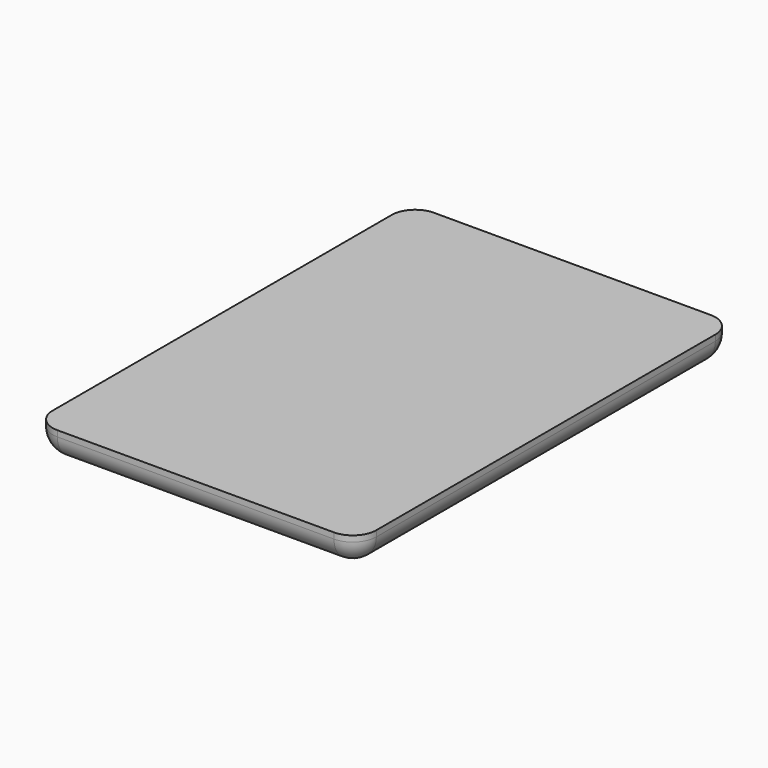
from build123d import *

# Parameters (mm, degrees)
F0_W         = 69.85
F0_H         = 101.6
F1_DEPTH     = 6.35
F2_R         = 5.08
F3_T1_DEPTH  = 13.97
F3_S5_W      = 5.08
F3_S5_H      = 5.08
F3_T6_DEPTH  = 5.08
F3_S11_W     = 5.08
F3_S11_H     = 5.08
F3_T12_DEPTH = 5.08
F3_S17_W     = 5.08
F3_S17_H     = 5.08
F3_T18_DEPTH = 5.08
F3_S23_W     = 5.08
F3_S23_H     = 5.08
F3_T24_DEPTH = 5.08


# Not quite as in the source:
# - a fillet or chamfer that OpenCascade refuses, or shapes differently, is made with other operations: its cross-section is extruded or revolved along the edge and cut away or added


with BuildPart() as f1:
    # F0 (on Top) → F1 (new body)
    with BuildSketch(Plane.XY):
        with Locations((34.925, -50.8)):
            Rectangle(F0_W, F0_H)
    extrude(amount=F1_DEPTH)

    # F2
    f2_edges = [f1.edges().sort_by_distance(p)[0] for p in [
        (69.85, -50.8, 0),
        (34.925, -101.6, 0),
        (0, -50.8, 0),
        (34.925, 0, 0),
    ]]
    fillet(f2_edges, radius=F2_R)

    # F3: fillet of radius 5.08 on 4 edges, made by hand

    # F3_s2 → F3_t1 (cut)
    with BuildSketch(Plane.XY.offset(5.08)):
        with BuildLine():
            ThreePointArc((0, -96.52), (1.4878975516, -100.1121024484), (5.08, -101.6))
            Line((5.08, -101.6), (0, -101.6))
            Line((0, -101.6), (0, -96.52))
        make_face()
        with BuildLine():
            ThreePointArc((64.77, 0), (68.3621024484, -1.4878975516), (69.85, -5.08))
            Line((69.85, -5.08), (69.85, 0))
            Line((69.85, 0), (64.77, 0))
        make_face()
        with BuildLine():
            ThreePointArc((5.08, 0), (1.4878975516, -1.4878975516), (0, -5.08))
            Line((0, -5.08), (0, 0))
            Line((0, 0), (5.08, 0))
        make_face()
        with BuildLine():
            ThreePointArc((69.85, -96.52), (68.3621024484, -100.1121024484), (64.77, -101.6))
            Line((64.77, -101.6), (69.85, -101.6))
            Line((69.85, -101.6), (69.85, -96.52))
        make_face()
    extrude(amount=F3_T1_DEPTH, mode=Mode.SUBTRACT)


with BuildPart() as f3_tool4:
    # F3_s5 → F3_t6 (new body)
    with BuildSketch(Plane.YZ.offset(64.77)):
        with Locations((-99.06, 2.54)):
            Rectangle(F3_S5_W, F3_S5_H)
    extrude(amount=F3_T6_DEPTH)

    # F3_s7 → F3_t8 (revolve, cut)
    with BuildSketch(Plane(origin=(64.77, -96.52, 5.08), x_dir=(0, 0.7071067812, 0.7071067812), z_dir=(0, 0.7071067812, -0.7071067812))):
        with BuildLine():
            ThreePointArc((0, -5.08), (5.08, 0), (0, 5.08))
            Line((0, 5.08), (0, -5.08))
        make_face()
    revolve(axis=Axis((64.77, -96.52, 5.08), (1, 0, 0)), mode=Mode.SUBTRACT)


with BuildPart() as f1_1:
    add(f1.part)

    # F3_t3: cut F3_tool4
    add(f3_tool4.part, mode=Mode.SUBTRACT)


with BuildPart() as f3_tool10:
    # F3_s11 → F3_t12 (new body)
    with BuildSketch(Plane.XZ.offset(5.08)):
        with Locations((2.54, 2.54)):
            Rectangle(F3_S11_W, F3_S11_H)
    extrude(amount=-F3_T12_DEPTH)

    # F3_s13 → F3_t14 (revolve, cut)
    with BuildSketch(Plane(origin=(5.08, -5.08, 5.08), x_dir=(0.7071067812, 0, 0.7071067812), z_dir=(-0.7071067812, 0, 0.7071067812))):
        with BuildLine():
            ThreePointArc((0, -5.08), (5.08, 0), (0, 5.08))
            Line((0, 5.08), (0, -5.08))
        make_face()
    revolve(axis=Axis((5.08, -5.08, 5.08), (0, 1, 0)), mode=Mode.SUBTRACT)


with BuildPart() as f1_2:
    add(f1_1.part)

    # F3_t9: cut F3_tool10
    add(f3_tool10.part, mode=Mode.SUBTRACT)


with BuildPart() as f3_tool16:
    # F3_s17 → F3_t18 (new body)
    with BuildSketch(Plane.XZ.offset(5.08)):
        with Locations((67.31, 2.54)):
            Rectangle(F3_S17_W, F3_S17_H)
    extrude(amount=-F3_T18_DEPTH)

    # F3_s19 → F3_t20 (revolve, cut)
    with BuildSketch(Plane(origin=(64.77, -5.08, 5.08), x_dir=(-0.7071067812, 0, 0.7071067812), z_dir=(-0.7071067812, 0, -0.7071067812))):
        with BuildLine():
            ThreePointArc((0, -5.08), (5.08, 0), (0, 5.08))
            Line((0, 5.08), (0, -5.08))
        make_face()
    revolve(axis=Axis((64.77, -5.08, 5.08), (0, 1, 0)), mode=Mode.SUBTRACT)


with BuildPart() as f1_3:
    add(f1_2.part)

    # F3_t15: cut F3_tool16
    add(f3_tool16.part, mode=Mode.SUBTRACT)


with BuildPart() as f3_tool22:
    # F3_s23 → F3_t24 (new body)
    with BuildSketch(Plane.YZ.offset(5.08)):
        with Locations((-99.06, 2.54)):
            Rectangle(F3_S23_W, F3_S23_H)
    extrude(amount=-F3_T24_DEPTH)

    # F3_s25 → F3_t26 (revolve, cut)
    with BuildSketch(Plane(origin=(5.08, -96.52, 5.08), x_dir=(0, 0.7071067812, 0.7071067812), z_dir=(0, -0.7071067812, 0.7071067812))):
        with BuildLine():
            ThreePointArc((0, -5.08), (5.08, 0), (0, 5.08))
            Line((0, 5.08), (0, -5.08))
        make_face()
    revolve(axis=Axis((5.08, -96.52, 5.08), (-1, 0, 0)), mode=Mode.SUBTRACT)


with BuildPart() as f1_4:
    add(f1_3.part)

    # F3_t21: cut F3_tool22
    add(f3_tool22.part, mode=Mode.SUBTRACT)


solid = f1_4.part
